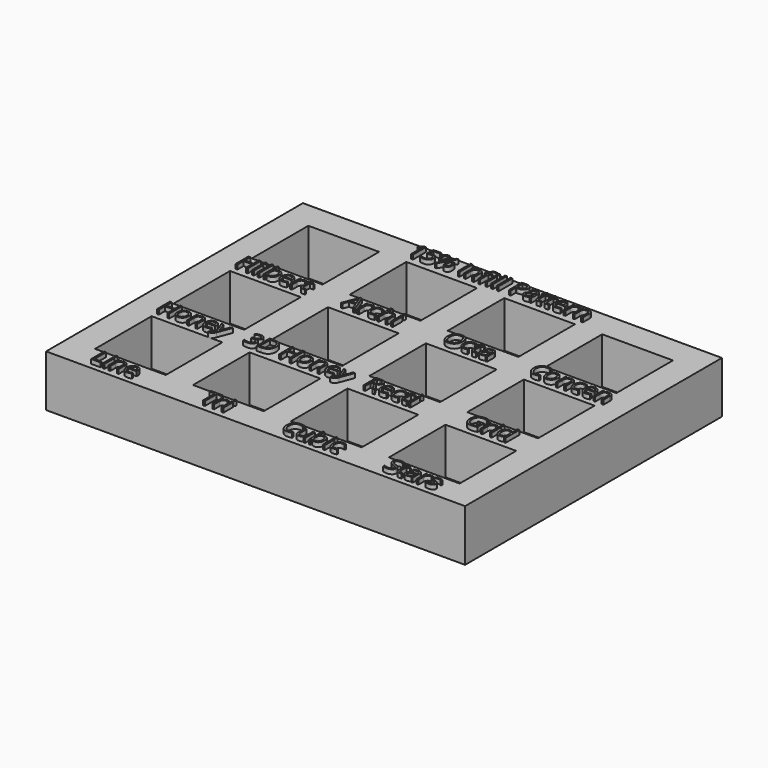
from build123d import *

# Parameters (mm, degrees)
F0_W         = 154
F0_H         = 118
F0_W_2       = 26
F0_H_2       = 26
F1_DEPTH     = 19
F2_DEPTH     = 17
F3_TEXT_SIZE = 8.3333333333
F4_DEPTH     = 1.6


# Not quite as in the source:
# - Text() gives the source's letters only with a copy of the font that has no kerning and outlines rounded to 1/6400 em; it was checked with that copy


with BuildPart() as f1:
    # F0 (on Top) → F1 (new body)
    with BuildSketch(Plane.XY):
        with Locations((-77, 59)):
            Rectangle(F0_W, F0_H)
        with Locations((-131, 23)):
            Rectangle(F0_W_2, F0_H_2, mode=Mode.SUBTRACT)
        with Locations((-95, 23)):
            Rectangle(F0_W_2, F0_H_2, mode=Mode.SUBTRACT)
        with Locations((-59, 23)):
            Rectangle(F0_W_2, F0_H_2, mode=Mode.SUBTRACT)
        with Locations((-23, 23)):
            Rectangle(F0_W_2, F0_H_2, mode=Mode.SUBTRACT)
        with Locations((-131, 59)):
            Rectangle(F0_W_2, F0_H_2, mode=Mode.SUBTRACT)
        with Locations((-95, 59)):
            Rectangle(F0_W_2, F0_H_2, mode=Mode.SUBTRACT)
        with Locations((-131, 95)):
            Rectangle(F0_W_2, F0_H_2, mode=Mode.SUBTRACT)
        with Locations((-95, 95)):
            Rectangle(F0_W_2, F0_H_2, mode=Mode.SUBTRACT)
        with Locations((-59, 59)):
            Rectangle(F0_W_2, F0_H_2, mode=Mode.SUBTRACT)
        with Locations((-23, 59)):
            Rectangle(F0_W_2, F0_H_2, mode=Mode.SUBTRACT)
        with Locations((-59, 95)):
            Rectangle(F0_W_2, F0_H_2, mode=Mode.SUBTRACT)
        with Locations((-23, 95)):
            Rectangle(F0_W_2, F0_H_2, mode=Mode.SUBTRACT)
        with Locations((-131, 23)):
            Rectangle(F0_W_2, F0_H_2)
        with Locations((-95, 23)):
            Rectangle(F0_W_2, F0_H_2)
        with Locations((-59, 23)):
            Rectangle(F0_W_2, F0_H_2)
        with Locations((-23, 23)):
            Rectangle(F0_W_2, F0_H_2)
        with Locations((-131, 59)):
            Rectangle(F0_W_2, F0_H_2)
        with Locations((-95, 59)):
            Rectangle(F0_W_2, F0_H_2)
        with Locations((-59, 59)):
            Rectangle(F0_W_2, F0_H_2)
        with Locations((-23, 59)):
            Rectangle(F0_W_2, F0_H_2)
        with Locations((-23, 95)):
            Rectangle(F0_W_2, F0_H_2)
        with Locations((-59, 95)):
            Rectangle(F0_W_2, F0_H_2)
        with Locations((-95, 95)):
            Rectangle(F0_W_2, F0_H_2)
        with Locations((-131, 95)):
            Rectangle(F0_W_2, F0_H_2)
    extrude(amount=-F1_DEPTH)

    # F0 (on Top) → F2 (cut)
    with BuildSketch(Plane.XY):
        with Locations((-131, 23)):
            Rectangle(F0_W_2, F0_H_2)
        with Locations((-95, 23)):
            Rectangle(F0_W_2, F0_H_2)
        with Locations((-59, 23)):
            Rectangle(F0_W_2, F0_H_2)
        with Locations((-23, 23)):
            Rectangle(F0_W_2, F0_H_2)
        with Locations((-131, 59)):
            Rectangle(F0_W_2, F0_H_2)
        with Locations((-95, 59)):
            Rectangle(F0_W_2, F0_H_2)
        with Locations((-23, 59)):
            Rectangle(F0_W_2, F0_H_2)
        with Locations((-23, 95)):
            Rectangle(F0_W_2, F0_H_2)
        with Locations((-59, 95)):
            Rectangle(F0_W_2, F0_H_2)
        with Locations((-95, 95)):
            Rectangle(F0_W_2, F0_H_2)
        with Locations((-131, 95)):
            Rectangle(F0_W_2, F0_H_2)
        with Locations((-59, 59)):
            Rectangle(F0_W_2, F0_H_2)
    extrude(amount=-F2_DEPTH, mode=Mode.SUBTRACT)

    # F3 (on face) → F4 (join)
    with BuildSketch(Plane.XY):
        with Locations((-110.3184148669, 110.3227520883)):
            Text('15% Infill Pattern', F3_TEXT_SIZE, font='Open Sans', text_align=(TextAlign.LEFT, TextAlign.BOTTOM))
        with Locations((-144.3888850742, 74)):
            Text('Hilbert', F3_TEXT_SIZE, font='Open Sans', text_align=(TextAlign.LEFT, TextAlign.BOTTOM))
        with Locations((-104.8788846103, 74)):
            Text('Archi', F3_TEXT_SIZE, font='Open Sans', text_align=(TextAlign.LEFT, TextAlign.BOTTOM))
        with Locations((-68.4956460843, 74)):
            Text('Octa', F3_TEXT_SIZE, font='Open Sans', text_align=(TextAlign.LEFT, TextAlign.BOTTOM))
        with Locations((-36.8558361249, 74)):
            Text('Concen', F3_TEXT_SIZE, font='Open Sans', text_align=(TextAlign.LEFT, TextAlign.BOTTOM))
        with Locations((-144.4708470239, 38)):
            Text('Honey', F3_TEXT_SIZE, font='Open Sans', text_align=(TextAlign.LEFT, TextAlign.BOTTOM))
        with Locations((-112.5750322408, 38)):
            Text('3D Honey', F3_TEXT_SIZE, font='Open Sans', text_align=(TextAlign.LEFT, TextAlign.BOTTOM))
        with Locations((-68.6049982905, 38)):
            Text('Recti', F3_TEXT_SIZE, font='Open Sans', text_align=(TextAlign.LEFT, TextAlign.BOTTOM))
        with Locations((-31.4683131874, 38)):
            Text('Grid', F3_TEXT_SIZE, font='Open Sans', text_align=(TextAlign.LEFT, TextAlign.BOTTOM))
        with Locations((-139.8207917809, 2)):
            Text('Line', F3_TEXT_SIZE, font='Open Sans', text_align=(TextAlign.LEFT, TextAlign.BOTTOM))
        with Locations((-99.8365730047, 2)):
            Text('Tri', F3_TEXT_SIZE, font='Open Sans', text_align=(TextAlign.LEFT, TextAlign.BOTTOM))
        with Locations((-70.0560435653, 2)):
            Text('Cubic', F3_TEXT_SIZE, font='Open Sans', text_align=(TextAlign.LEFT, TextAlign.BOTTOM))
        with Locations((-32.3261171579, 2)):
            Text('Stars', F3_TEXT_SIZE, font='Open Sans', text_align=(TextAlign.LEFT, TextAlign.BOTTOM))
    extrude(amount=F4_DEPTH)


solid = f1.part
